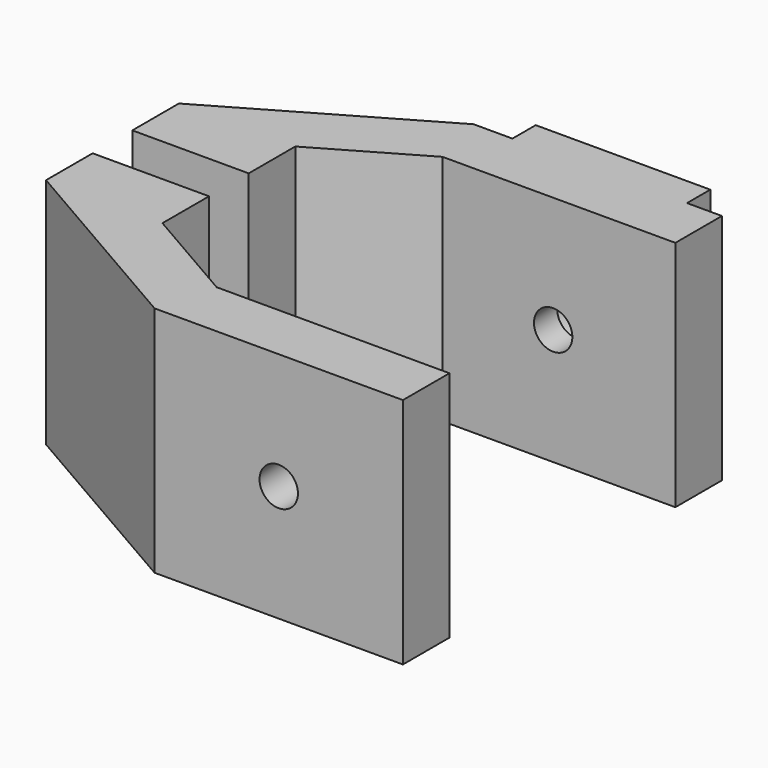
from build123d import *

# Parameters (mm, degrees)
F0_W     = 10
F0_H     = 5
F1_DEPTH = 20
F2_R     = 3.05
F3_DEPTH = 5
F4_R     = 1.65
F5_DEPTH = 31.7638052831
F6_R     = 1.65
F7_DEPTH = 36.7638052831


with BuildPart() as f1:
    # F0 (on Top) → F1 (new body)
    with BuildSketch(Plane.XY):
        Rectangle(F0_W, F0_H)
        Polygon((-5, 2.5), (5, 2.5), (13.6602540378, 7.5), (33.6602540378, 7.5), (33.6602540378, 12.5), (30.6602540378, 12.5), (24.6622947636, 12.5), (15.6602540378, 12.5), (12.3205080757, 12.5), align=None)
        Polygon((15.6602540378, 15), (15.6602540378, 12.5), (24.6622947636, 12.5), (30.6602540378, 12.5), (30.6602540378, 15), align=None)
    extrude(amount=F1_DEPTH)

    # F2 (on face) → F3 (cut)
    with BuildSketch(Plane(origin=(0, 15, 0), x_dir=(-1, 0, 0), z_dir=(0, 1, 0))):
        with Locations((-23.1602540378, 10)):
            Circle(F2_R)
    extrude(amount=-F3_DEPTH, mode=Mode.SUBTRACT)

    # F4 (on face) → F5 (cut, through all)
    with BuildSketch(Plane(origin=(0, 10, 0), x_dir=(-1, 0, 0), z_dir=(0, 1, 0))):
        with Locations((-23.1602540378, 10)):
            Circle(F4_R)
    extrude(amount=-F5_DEPTH, mode=Mode.SUBTRACT)


with BuildPart() as f1b:
    # F0 (on Top) → F1, piece 2 (new body)
    with BuildSketch(Plane.XY):
        with Locations((0, -9.2628052831)):
            Rectangle(F0_W, F0_H)
        Polygon((5, -11.7628052831), (-5, -11.7628052831), (12.3205080757, -21.7628052831), (33.6602540378, -21.7628052831), (33.6602540378, -16.7628052831), (13.6602540378, -16.7628052831), align=None)
    extrude(amount=F1_DEPTH)

    # F6 (on face) → F7 (cut, through all)
    with BuildSketch(Plane.XZ.offset(21.7628052831)):
        with Locations((22.9903810568, 10)):
            Circle(F6_R)
    extrude(amount=-F7_DEPTH, mode=Mode.SUBTRACT)


solid = Compound([f1.part, f1b.part])
